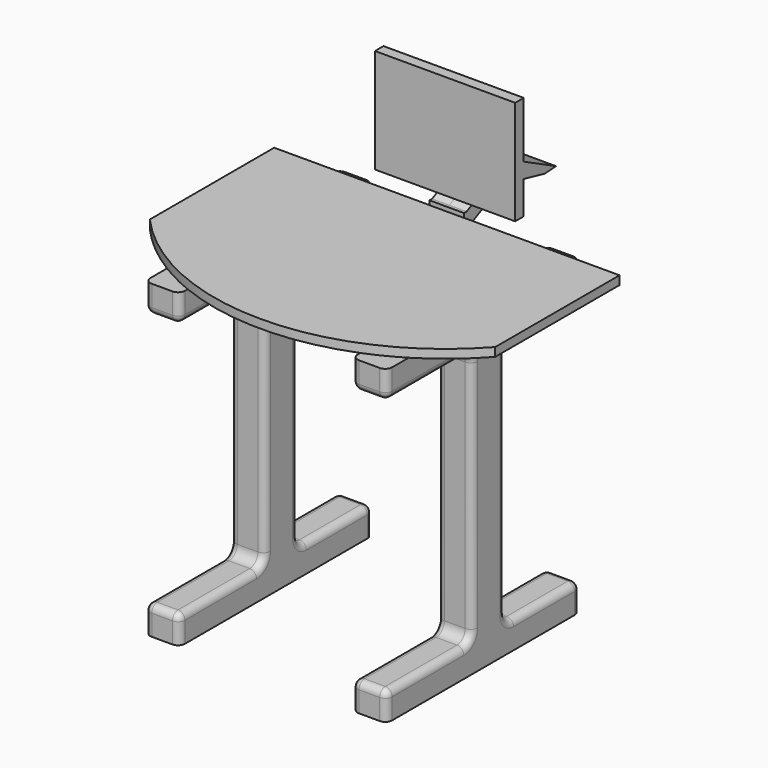
from build123d import *

# Parameters (mm, degrees)
F1_DEPTH = 900
F3_DEPTH = 25
F5_DEPTH = 759
F7_DEPTH = 50
F9_DEPTH = 203
F10_R    = 20


# Not quite as in the source:
# - the dataset's text gives a spline's control points without its knots; the knots are read off the source's solid


with BuildPart() as f1:
    # F0 (on Top) → F1 (new body)
    with BuildSketch(Plane.XY):
        with BuildLine():
            Line((270, -301.3999864981), (330, -301.3999864981))
            ThreePointArc((330, -301.3999864981), (344.1421356237, -295.5421221218), (350, -281.3999864981))
            Line((350, -281.3999864981), (350, 378.6000135019))
            ThreePointArc((350, 378.6000135019), (344.1421356237, 392.7421491256), (330, 398.6000135019))
            Line((330, 398.6000135019), (270, 398.6000135019))
            ThreePointArc((270, 398.6000135019), (255.8578643763, 392.7421491256), (250, 378.6000135019))
            Line((250, 378.6000135019), (250, -281.3999864981))
            ThreePointArc((250, -281.3999864981), (255.8578643763, -295.5421221218), (270, -301.3999864981))
        make_face()
    extrude(amount=F1_DEPTH)



with BuildPart() as f1b:
    # F0 (on Top) → F1, piece 2 (new body)
    with BuildSketch(Plane.XY):
        with BuildLine():
            Line((-270, 398.6000135019), (-330, 398.6000135019))
            ThreePointArc((-330, 398.6000135019), (-344.1421356237, 392.7421491256), (-350, 378.6000135019))
            Line((-350, 378.6000135019), (-350, -281.3999864981))
            ThreePointArc((-350, -281.3999864981), (-344.1421356237, -295.5421221218), (-330, -301.3999864981))
            Line((-330, -301.3999864981), (-270, -301.3999864981))
            ThreePointArc((-270, -301.3999864981), (-255.8578643763, -295.5421221218), (-250, -281.3999864981))
            Line((-250, -281.3999864981), (-250, 378.6000135019))
            ThreePointArc((-250, 378.6000135019), (-255.8578643763, 392.7421491256), (-270, 398.6000135019))
        make_face()
    extrude(amount=F1_DEPTH)


with BuildPart() as f1_1:
    add(f1.part)

    add(f1b.part)  # F3 merges F1b
    # F2 (on face) → F3 (join)
    with BuildSketch(Plane.XY.offset(900)):
        with BuildLine():
            Line((500, 354.0968874406), (0, 354.0968874406))
            Line((0, 354.0968874406), (-500, 354.0968874406))
            Line((-500, 354.0968874406), (-500, -95.9031125594))
            ThreePointArc((-500, -95.9031125594), (0, -319.9657073101), (500, -95.9031125594))
            Line((500, -95.9031125594), (500, 354.0968874406))
        make_face()
    extrude(amount=F3_DEPTH)

    # F4 (on face) → F5 (cut)
    with BuildSketch(Plane.YZ.offset(350)):
        with BuildLine():
            Line((-21.994241029, 819.2238211632), (-362.487912178, 819.2238211632))
            Line((-362.487912178, 819.2238211632), (-362.487912178, 80.0541564822))
            Line((-362.487912178, 80.0541564822), (-21.994241029, 80.0541564822))
            ThreePointArc((-21.994241029, 80.0541564822), (-0.7810375934, 88.8409530466), (8.005758971, 110.0541564822))
            Line((8.005758971, 110.0541564822), (8.005758971, 789.2238211632))
            ThreePointArc((8.005758971, 789.2238211632), (-0.7810375934, 810.4370245988), (-21.994241029, 819.2238211632))
        make_face()
        with BuildLine():
            Line((498.7023770809, 80.0541564822), (498.7023770809, 819.2238211632))
            Line((498.7023770809, 819.2238211632), (158.2087059319, 819.2238211632))
            ThreePointArc((158.2087059319, 819.2238211632), (136.9955024963, 810.4370245988), (128.2087059319, 789.2238211632))
            Line((128.2087059319, 789.2238211632), (128.2087059319, 110.0541564822))
            ThreePointArc((128.2087059319, 110.0541564822), (136.9955024963, 88.8409530466), (158.2087059319, 80.0541564822))
            Line((158.2087059319, 80.0541564822), (498.7023770809, 80.0541564822))
        make_face()
    extrude(amount=-F5_DEPTH, mode=Mode.SUBTRACT)

    # F6 (on Right) → F7 (join, symmetric)
    with BuildSketch(Plane.YZ):
        with BuildLine():
            Line((353.656232357, 901.1268019676), (379.8283934593, 901.1268019676))
            add(Edge.make_bspline(
                [(379.8283934593, 901.1268019676), (422.3837230355, 920.7091528548), (499.6166790446, 956.2488340106), (495.6051130218, 1020.7542373892), (493.8039183617, 1049.7171878815)],
                knots=[0, 0, 0, 0, 0.5509996221, 1, 1, 1, 1], degree=3))
            Line((493.8039183617, 1049.7171878815), (453.8810456708, 1047.2343999097))
            add(Edge.make_bspline(
                [(363.1073069511, 937.4641830783), (367.9343667017, 939.6854131506), (377.4672104241, 944.0724360889), (391.1779254464, 950.5529507421), (404.0577618072, 956.9762611694), (415.8472252163, 963.3544576802), (424.5344200434, 968.6067253019), (430.6634256366, 972.7220805755), (434.8173528204, 975.7443355216), (438.499282352, 978.6764659525), (441.6862358998, 981.4858336752), (444.3651641507, 984.1344123192), (446.1752123772, 986.1731652397), (447.3807636814, 987.6844011884), (448.1684393344, 988.7537266092), (448.7341126413, 989.5911280023), (449.1335016109, 990.2239588168), (449.5208403617, 990.8677971689), (449.9819329197, 991.6927062968), (450.6787671472, 993.0710893782), (451.4825722447, 994.9286693816), (452.3517667196, 997.4427065704), (453.1197689804, 1000.29033594), (453.77288069, 1003.4991162269), (454.4716498579, 1008.2701417785), (454.9920392912, 1015.1474588944), (455.0411601437, 1024.7191842146), (454.6141334, 1035.4222883151), (454.1317685473, 1043.2028121986), (453.8810456708, 1047.2343999097)],
                knots=[0, 0, 0, 0, 0.0625, 0.125, 0.1875, 0.25, 0.3125, 0.34375, 0.375, 0.40625, 0.4375, 0.46875, 0.5, 0.515625, 0.53125, 0.546875, 0.5546875, 0.5625, 0.578125, 0.59375, 0.625, 0.65625, 0.6875, 0.71875, 0.75, 0.8125, 0.875, 0.9375, 1, 1, 1, 1], degree=3))
            Line((363.1073069511, 937.4641830783), (353.656232357, 937.4641830783))
            Line((353.656232357, 937.4641830783), (353.656232357, 901.1268019676))
        make_face()
    extrude(amount=F7_DEPTH, both=True)

    # F8 (on Right) → F9 (join, symmetric)
    with BuildSketch(Plane.YZ):
        Polygon((347.6943671703, 968.5171246529), (378.5805404186, 968.5171246529), (378.5805404186, 1063.8613700867), (378.5805404186, 1108.1763505936), (378.5805404186, 1270.6644535065), (347.6943671703, 1270.6644535065), align=None)
        Polygon((378.5805404186, 1108.1763505936), (378.5805404186, 1063.8613700867), (455.124527216, 1046.404004097), (495.4108297825, 1049.0897893906), align=None)
    extrude(amount=F9_DEPTH, both=True)

    # F10
    f10_edges = [f1_1.edges().sort_by_distance(p)[0] for p in [
        (350, -151.697114, 80.054156),
        (-250, -151.697114, 80.054156),
        (-350, 268.40436, 80.054156),
        (250, 268.40436, 80.054156),
        (-300, -301.399986, 80.054156),
        (-255.857864, -295.542122, 80.054156),
        (-350, -151.697114, 80.054156),
        (-344.142136, -295.542122, 80.054156),
        (-250, 268.40436, 80.054156),
        (-250, 136.995502, 88.840953),
        (-250, 128.208706, 449.638989),
        (-250, 136.995502, 810.437025),
        (-250, 268.40436, 819.223821),
        (-250, -151.697114, 819.223821),
        (-250, -0.781038, 810.437025),
        (-250, 8.005759, 449.638989),
        (-250, -0.781038, 88.840953),
        (-255.857864, 392.742149, 80.054156),
        (-300, 398.600014, 80.054156),
        (-344.142136, 392.742149, 80.054156),
        (-350, -0.781038, 88.840953),
        (-350, 8.005759, 449.638989),
        (-350, -0.781038, 810.437025),
        (-350, -151.697114, 819.223821),
        (-350, 268.40436, 819.223821),
        (-350, 136.995502, 810.437025),
        (-350, 128.208706, 449.638989),
        (-350, 136.995502, 88.840953),
        (-344.142136, 392.742149, 819.223821),
        (-300, 398.600014, 819.223821),
        (-255.857864, 392.742149, 819.223821),
        (-255.857864, -295.542122, 819.223821),
        (-300, -301.399986, 819.223821),
        (-344.142136, -295.542122, 819.223821),
        (250, -151.697114, 80.054156),
        (250, -0.781038, 88.840953),
        (250, 8.005759, 449.638989),
        (250, -0.781038, 810.437025),
        (250, -151.697114, 819.223821),
        (250, 268.40436, 819.223821),
        (250, 136.995502, 810.437025),
        (250, 128.208706, 449.638989),
        (250, 136.995502, 88.840953),
        (255.857864, -295.542122, 80.054156),
        (300, -301.399986, 80.054156),
        (344.142136, -295.542122, 80.054156),
        (350, -0.781038, 88.840953),
        (350, 8.005759, 449.638989),
        (350, -0.781038, 810.437025),
        (350, -151.697114, 819.223821),
        (344.142136, -295.542122, 819.223821),
        (300, -301.399986, 819.223821),
        (255.857864, -295.542122, 819.223821),
        (255.857864, 392.742149, 819.223821),
        (350, 268.40436, 819.223821),
        (300, 398.600014, 819.223821),
        (344.142136, 392.742149, 819.223821),
        (350, 136.995502, 810.437025),
        (350, 128.208706, 449.638989),
        (350, 136.995502, 88.840953),
        (350, 268.40436, 80.054156),
        (344.142136, 392.742149, 80.054156),
        (300, 398.600014, 80.054156),
        (255.857864, 392.742149, 80.054156),
    ]]
    fillet(f10_edges, radius=F10_R)


solid = f1_1.part
